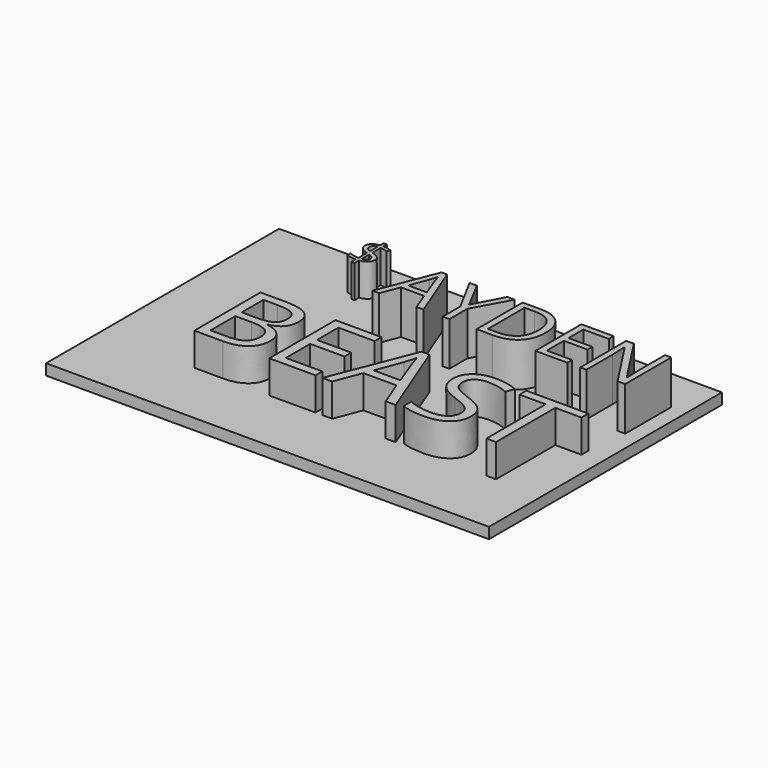
from build123d import *

# Parameters (mm, degrees)
F0_TEXT_SIZE = 67.2911138584
F1_DEPTH     = 25.4
F2_TEXT_SIZE = 28.7082615412
F3_DEPTH     = 25.4
F4_W         = 257.3693171144
F4_H         = 169.2382395267
F5_DEPTH     = 6.35
F6_TEXT_SIZE = 46.8652422975
F7_DEPTH     = 25.4


# Not quite as in the source:
# - Text() gives the source's letters only with a copy of the font that has no kerning and outlines rounded to 1/6400 em; it was checked with that copy


with BuildPart() as f1:
    # F0 (on Top) → F1 (new body)
    with BuildSketch(Plane.XY):
        with Locations((-55.9575110674, -48.4496019781)):
            Text('BEAST', F0_TEXT_SIZE, font='Open Sans', text_align=(TextAlign.LEFT, TextAlign.BOTTOM))
    extrude(amount=F1_DEPTH)


with BuildPart() as f3:
    # F2 (on Top) → F3 (new body)
    with BuildSketch(Plane.XY):
        with Locations((-43.181322515, 50.5036525428)):
            Text('$', F2_TEXT_SIZE, font='Open Sans', text_align=(TextAlign.LEFT, TextAlign.BOTTOM))
    extrude(amount=F3_DEPTH)


with BuildPart() as f5:
    # F4 (on Top) → F5 (new body)
    with BuildSketch(Plane.XY):
        with Locations((23.9673219621, -2.3166835308)):
            Rectangle(F4_W, F4_H)
    extrude(amount=F5_DEPTH)

    # F6 (on face) → F7 (join)
    with BuildSketch(Plane.XY.offset(6.35)):
        with Locations((-3.1173365951, 23.1594617784)):
            Text('AYDEN', F6_TEXT_SIZE, font='Open Sans', text_align=(TextAlign.LEFT, TextAlign.BOTTOM))
    extrude(amount=F7_DEPTH)


solid = Compound([f1.part, f3.part, f5.part])
